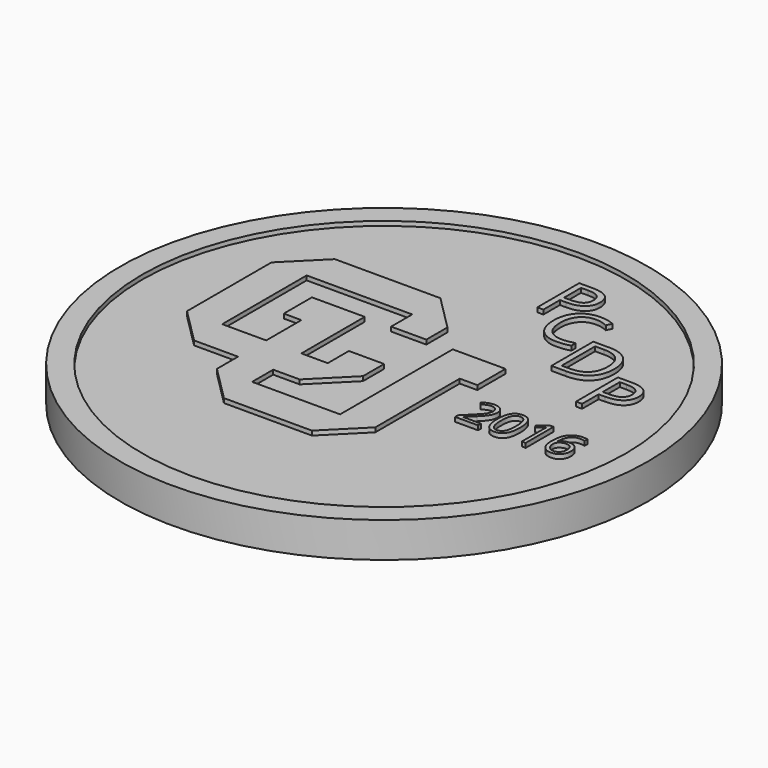
from build123d import *

# Parameters (mm, degrees)
F0_R           = 38.1
F1_DEPTH       = 3.81
F2_R           = 38.1
F2_R_2         = 34.925
F2_TEXT_SIZE   = 10.5833333333
F2_TEXT_SIZE_2 = 7.0555555556
F3_DEPTH       = 0.635
F4_R           = 38.1
F4_R_2         = 34.925
F4_TEXT_SIZE   = 10.5833333333
F4_R_3         = 2.54
F4_R_4         = 0.635
F5_DEPTH       = 0.635


# Not quite as in the source:
# - Text() gives the source's letters only with a copy of the font that has no kerning and outlines rounded to 1/6400 em; it was checked with that copy


with BuildPart() as f1:
    # F0 (on Top) → F1 (new body)
    with BuildSketch(Plane.XY):
        Circle(F0_R)
    extrude(amount=F1_DEPTH)

    # F2 (on face) → F3 (join)
    with BuildSketch(Plane.XY.offset(3.81)):
        Circle(F2_R)
        Circle(F2_R_2, mode=Mode.SUBTRACT)
        with Locations((3.81, 21.59)):
            Text('P', F2_TEXT_SIZE, font='Open Sans', text_align=(TextAlign.LEFT, TextAlign.BOTTOM))
        with Locations((7.62, 16.51)):
            Text('C', F2_TEXT_SIZE, font='Open Sans', text_align=(TextAlign.LEFT, TextAlign.BOTTOM))
        with Locations((13.97, 11.43)):
            Text('D', F2_TEXT_SIZE, font='Open Sans', text_align=(TextAlign.LEFT, TextAlign.BOTTOM))
        with Locations((21.59, 6.35)):
            Text('P', F2_TEXT_SIZE, font='Open Sans', text_align=(TextAlign.LEFT, TextAlign.BOTTOM))
        Polygon((0, -3.81), (0, 0), (-5.08, 0), (-5.08, -3.81), (-8.89, -3.81), (-8.89, 7.62), (-16.51, 7.62), (-16.51, 2.54), (-13.97, 2.54), (-13.97, -3.81), (-20.32, -3.81), (-20.32, 11.43), (-5.08, 11.43), (-5.08, 7.62), (0, 7.62), (0, 11.43), (-5.08, 16.51), (-20.32, 16.51), (-25.4, 11.43), (-25.4, -3.81), (-20.32, -8.89), (-13.97, -8.89), (-13.97, -12.7), (-8.89, -17.78), (3.81, -17.78), (8.89, -12.7), (8.89, 2.54), (11.43, 2.54), (11.43, 7.62), (3.81, 7.62), (3.81, -12.7), (-8.89, -12.7), (-8.89, -8.89), (-5.08, -8.89), align=None)
        with Locations((13.97, -5.08)):
            Text('2016', F2_TEXT_SIZE_2, font='Open Sans', text_align=(TextAlign.LEFT, TextAlign.BOTTOM))
    extrude(amount=F3_DEPTH)

    # F4 (on face) → F5 (join)
    with BuildSketch(Plane(origin=(0, 0, 0), x_dir=(1, 0, 0), z_dir=(0, 0, -1))):
        Circle(F4_R)
        Circle(F4_R_2, mode=Mode.SUBTRACT)
        with Locations((-12.709921875, 19.05)):
            Text('Chris', F4_TEXT_SIZE, font='Open Sans', text_align=(TextAlign.LEFT, TextAlign.BOTTOM))
        with BuildLine():
            Line((4.8866127978, 13.4258583195), (5.4295697753, 14.917620355))
            ThreePointArc((5.4295697753, 14.917620355), (0, 15.875), (-5.4295697753, 14.917620355))
            Line((-5.4295697753, 14.917620355), (-4.8866127978, 13.4258583195))
            ThreePointArc((-4.8866127978, 13.4258583195), (-2.7931391001, 14.0118175201), (-0.635, 14.2733819135))
            Line((-0.635, 14.2733819135), (-0.635, 11.4123474798))
            ThreePointArc((-0.635, 11.4123474798), (-5.715, 9.8986703653), (-9.5658828343, 6.2560998713))
            Line((-9.5658828343, 6.2560998713), (-12.043611335, 7.6866170882))
            ThreePointArc((-12.043611335, 7.6866170882), (-10.7380203755, 9.4248381771), (-9.1838279734, 10.9448599811))
            Line((-9.1838279734, 10.9448599811), (-10.2042533038, 12.1609555345))
            ThreePointArc((-10.2042533038, 12.1609555345), (-13.7481532851, 7.9375), (-15.6338230791, 2.7566648205))
            Line((-15.6338230791, 2.7566648205), (-14.0704407712, 2.4809983384))
            ThreePointArc((-14.0704407712, 2.4809983384), (-13.5311594757, 4.586979343), (-12.678611335, 6.5867648254))
            Line((-12.678611335, 6.5867648254), (-10.2008828343, 5.1562476085))
            ThreePointArc((-10.2008828343, 5.1562476085), (-11.43, 0), (-10.2008828343, -5.1562476085))
            Line((-10.2008828343, -5.1562476085), (-12.678611335, -6.5867648254))
            ThreePointArc((-12.678611335, -6.5867648254), (-13.5311594757, -4.586979343), (-14.0704407712, -2.4809983384))
            Line((-14.0704407712, -2.4809983384), (-15.6338230791, -2.7566648205))
            ThreePointArc((-15.6338230791, -2.7566648205), (-13.7481532851, -7.9375), (-10.2042533038, -12.1609555345))
            Line((-10.2042533038, -12.1609555345), (-9.1838279734, -10.9448599811))
            ThreePointArc((-9.1838279734, -10.9448599811), (-10.7380203755, -9.4248381771), (-12.043611335, -7.6866170882))
            Line((-12.043611335, -7.6866170882), (-9.5658828343, -6.2560998713))
            ThreePointArc((-9.5658828343, -6.2560998713), (-5.715, -9.8986703653), (-0.635, -11.4123474798))
            Line((-0.635, -11.4123474798), (-0.635, -14.2733819135))
            ThreePointArc((-0.635, -14.2733819135), (-2.7931391001, -14.0118175201), (-4.8866127978, -13.4258583195))
            Line((-4.8866127978, -13.4258583195), (-5.4295697753, -14.917620355))
            ThreePointArc((-5.4295697753, -14.917620355), (0, -15.875), (5.4295697753, -14.917620355))
            Line((5.4295697753, -14.917620355), (4.8866127978, -13.4258583195))
            ThreePointArc((4.8866127978, -13.4258583195), (2.7931391001, -14.0118175201), (0.635, -14.2733819135))
            Line((0.635, -14.2733819135), (0.635, -11.4123474798))
            ThreePointArc((0.635, -11.4123474798), (5.715, -9.8986703653), (9.5658828343, -6.2560998713))
            Line((9.5658828343, -6.2560998713), (12.043611335, -7.6866170882))
            ThreePointArc((12.043611335, -7.6866170882), (10.7380203755, -9.4248381771), (9.1838279734, -10.9448599811))
            Line((9.1838279734, -10.9448599811), (10.2042533038, -12.1609555345))
            ThreePointArc((10.2042533038, -12.1609555345), (13.7481532851, -7.9375), (15.6338230791, -2.7566648205))
            Line((15.6338230791, -2.7566648205), (14.0704407712, -2.4809983384))
            ThreePointArc((14.0704407712, -2.4809983384), (13.5311594757, -4.586979343), (12.678611335, -6.5867648254))
            Line((12.678611335, -6.5867648254), (10.2008828343, -5.1562476085))
            ThreePointArc((10.2008828343, -5.1562476085), (11.43, 0), (10.2008828343, 5.1562476085))
            Line((10.2008828343, 5.1562476085), (12.678611335, 6.5867648254))
            ThreePointArc((12.678611335, 6.5867648254), (13.5311594757, 4.586979343), (14.0704407712, 2.4809983384))
            Line((14.0704407712, 2.4809983384), (15.6338230791, 2.7566648205))
            ThreePointArc((15.6338230791, 2.7566648205), (13.7481532851, 7.9375), (10.2042533038, 12.1609555345))
            Line((10.2042533038, 12.1609555345), (9.1838279734, 10.9448599811))
            ThreePointArc((9.1838279734, 10.9448599811), (10.7380203755, 9.4248381771), (12.043611335, 7.6866170882))
            Line((12.043611335, 7.6866170882), (9.5658828343, 6.2560998713))
            ThreePointArc((9.5658828343, 6.2560998713), (5.715, 9.8986703653), (0.635, 11.4123474798))
            Line((0.635, 11.4123474798), (0.635, 14.2733819135))
            ThreePointArc((0.635, 14.2733819135), (2.7931391001, 14.0118175201), (4.8866127978, 13.4258583195))
        make_face()
        with BuildLine():
            Line((-5.7485135605, -8.3773618666), (-5.7485135605, -2.4884440919))
            ThreePointArc((-5.7485135605, -2.4884440919), (-4.3558129905, -2.7129720366), (-2.9545135605, -2.8754145889))
            Line((-2.9545135605, -2.8754145889), (-2.9545135605, -9.7209284341))
            ThreePointArc((-2.9545135605, -9.7209284341), (-4.4030629166, -9.1563440822), (-5.7485135605, -8.3773618666))
        make_face(mode=Mode.SUBTRACT)
        with BuildLine():
            ThreePointArc((-7.0185135605, -7.3461600446), (-9.0491945672, -4.6192724195), (-10.0665135605, -1.3751017185))
            ThreePointArc((-10.0665135605, -1.3751017185), (-8.5531444027, -1.8394166235), (-7.0185135605, -2.2277241263))
            Line((-7.0185135605, -2.2277241263), (-7.0185135605, -7.3461600446))
        make_face(mode=Mode.SUBTRACT)
        with BuildLine():
            Line((-1.6845135605, -10.0193819203), (-1.6845135605, -2.9684625287))
            ThreePointArc((-1.6845135605, -2.9684625287), (0, -3.0131804126), (1.6845135605, -2.9684625287))
            Line((1.6845135605, -2.9684625287), (1.6845135605, -10.0193819203))
            ThreePointArc((1.6845135605, -10.0193819203), (0, -10.16), (-1.6845135605, -10.0193819203))
        make_face(mode=Mode.SUBTRACT)
        with BuildLine():
            Line((2.9545135605, -9.7209284341), (2.9545135605, -2.8754145889))
            ThreePointArc((2.9545135605, -2.8754145889), (4.3558129905, -2.7129720366), (5.7485135605, -2.4884440919))
            Line((5.7485135605, -2.4884440919), (5.7485135605, -8.3773618666))
            ThreePointArc((5.7485135605, -8.3773618666), (4.4030629166, -9.1563440822), (2.9545135605, -9.7209284341))
        make_face(mode=Mode.SUBTRACT)
        with BuildLine():
            Line((7.0185135605, -7.3461600446), (7.0185135605, -2.2277241263))
            ThreePointArc((7.0185135605, -2.2277241263), (8.5531444027, -1.8394166235), (10.0665135605, -1.3751017185))
            ThreePointArc((10.0665135605, -1.3751017185), (9.0491945672, -4.6192724195), (7.0185135605, -7.3461600446))
        make_face(mode=Mode.SUBTRACT)
        with BuildLine():
            ThreePointArc((10.16, 0), (0, -1.7431804126), (-10.16, 0))
            ThreePointArc((-10.16, 0), (0, 10.16), (10.16, 0))
        make_face(mode=Mode.SUBTRACT)
        with Locations((4.572, 3.048)):
            Circle(F4_R_3)
        with Locations((-4.572, 3.048)):
            Circle(F4_R_3)
        Circle(F4_R_4)
        with Locations((-17.6286914063, -26.67)):
            Text('Choate', F4_TEXT_SIZE, font='Open Sans', text_align=(TextAlign.LEFT, TextAlign.BOTTOM))
    extrude(amount=F5_DEPTH)


solid = f1.part
